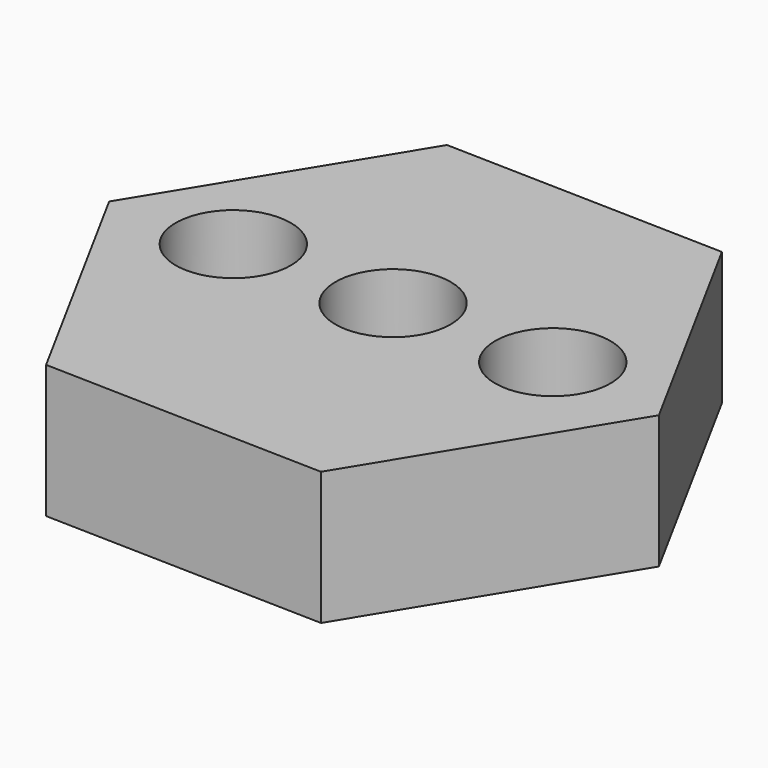
from build123d import *

# Parameters (mm, degrees)
F0_R     = 10.9855
F1_DEPTH = 25.4


# Not quite as in the source:
# - a feature names something its author has since deleted; it is built from what else it names


with BuildPart() as f1:
    # F0 (on Top) → F1 (new body)
    with BuildSketch(Plane.XY):
        Polygon((53.519200738, -3.5098091407), (27.9298310918, 43.5148113115), (-25.5893696461, 44.8660773572), (-53.519200738, -0.8072770493), (-27.9298310918, -47.8318975015), (25.5893696461, -49.1831635472), align=None)
        with Locations((-30.48, 0)):
            Circle(F0_R, mode=Mode.SUBTRACT)
        with BuildLine():
            ThreePointArc((-10.9855, 0), (0, 10.9855), (10.9855, 0))
            ThreePointArc((10.9855, 0), (0, -10.9855), (-10.9855, 0))
        make_face(mode=Mode.SUBTRACT)
        with BuildLine():
            ThreePointArc((41.4655, 0), (30.48, -10.9855), (19.4945, 0))
            ThreePointArc((19.4945, 0), (30.48, 10.9855), (41.4655, 0))
        make_face(mode=Mode.SUBTRACT)
    extrude(amount=F1_DEPTH)


solid = f1.part
